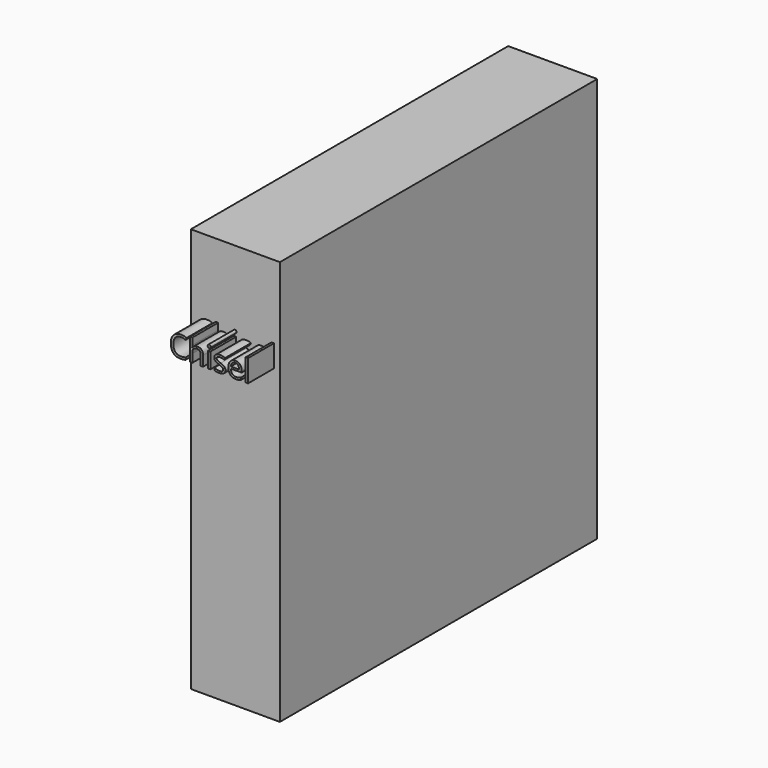
from build123d import *

# Parameters (mm, degrees)
F0_W         = 69.85
F0_H         = 317.5
F1_DEPTH     = 311.15
F2_TEXT_SIZE = 22.9436007452
F3_DEPTH     = 25.4


# Not quite as in the source:
# - Text() gives the source's letters only with a copy of the font that has no kerning and outlines rounded to 1/6400 em; it was checked with that copy


with BuildPart() as f1:
    # F0 (on Front) → F1 (new body)
    with BuildSketch(Plane.XZ):
        Rectangle(F0_W, F0_H)
    extrude(amount=F1_DEPTH)

    # F2 (on face) → F3 (join)
    with BuildSketch(Plane.XZ.offset(311.15)):
        with Locations((-31.75, 83.8264483354)):
            Text('Chisel', F2_TEXT_SIZE, font='Open Sans', text_align=(TextAlign.LEFT, TextAlign.BOTTOM))
    extrude(amount=F3_DEPTH)


solid = f1.part
